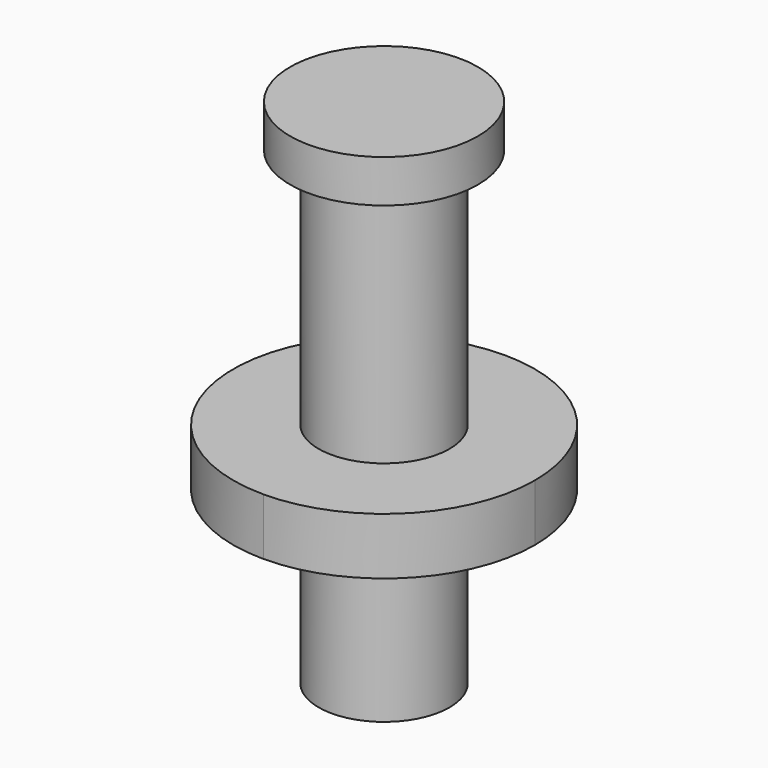
from build123d import *

# Parameters (mm, degrees)
F0_R          = 3.3
F0_R_2        = 2.3
F1_DEPTH      = 2
F2_DEPTH      = 10
F2_DEPTH_BACK = 8
F3_START      = 8.5
F3_DEPTH      = 1.5


with BuildPart() as f1:
    # F0 (on Top) → F1 (new body)
    with BuildSketch(Plane.XY):
        with BuildLine():
            ThreePointArc((-2.2, 0), (-3.7523340597, 3.7476659403), (-7.5, 5.3))
            ThreePointArc((-7.5, 5.3), (-12.8, 0), (-7.5, -5.3))
            ThreePointArc((-7.5, -5.3), (-3.7523340597, -3.7476659403), (-2.2, 0))
        make_face()
        with Locations((-7.5, 0)):
            Circle(F0_R, mode=Mode.SUBTRACT)
        with Locations((-7.5, 0)):
            Circle(F0_R)
        with Locations((-7.5, 0)):
            Circle(F0_R_2, mode=Mode.SUBTRACT)
    extrude(amount=-F1_DEPTH)

    # F0 (on Top) → F2 (join, two sides)
    with BuildSketch(Plane.XY) as f2_sk:
        with Locations((-7.5, 0)):
            Circle(F0_R_2)
    extrude(amount=F2_DEPTH)
    extrude(f2_sk.sketch, amount=-F2_DEPTH_BACK)

    # F0 (on Top) → F3 (join)
    with BuildSketch(Plane.XY.offset(F3_START)):
        with Locations((-7.5, 0)):
            Circle(F0_R)
        with Locations((-7.5, 0)):
            Circle(F0_R_2, mode=Mode.SUBTRACT)
    extrude(amount=F3_DEPTH)


solid = f1.part
